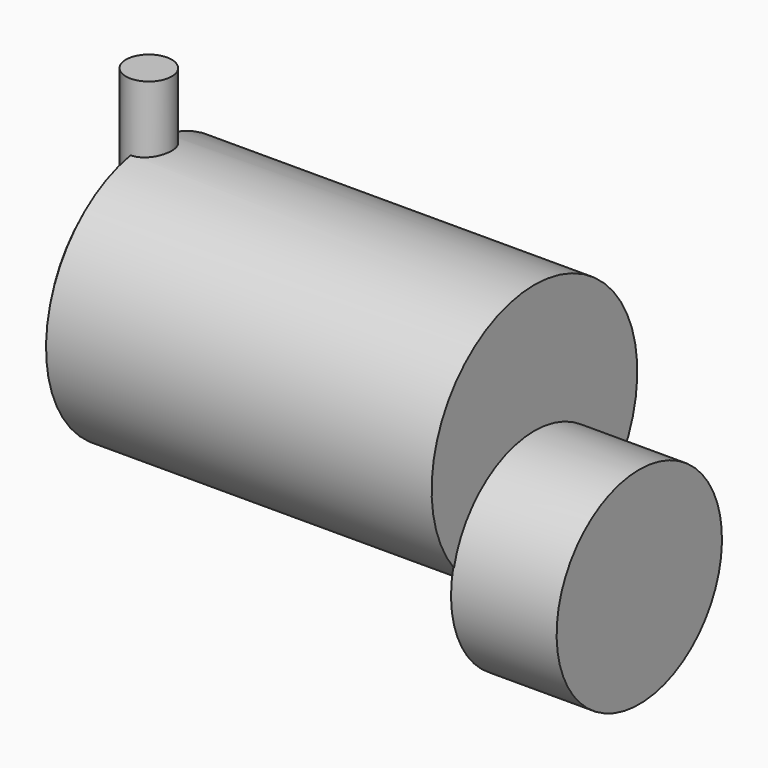
from build123d import *

# Parameters (mm, degrees)
F2_W = 54.2633533478
F2_H = 228.2263338566
F0_W = 914.4
F0_H = 304.8


# Not quite as in the source:
# - a feature names something its author has since deleted; it is built from what else it names


with BuildPart() as f3:
    # F2 (on Right) → F3 (revolve)
    with BuildSketch(Plane.YZ):
        with Locations((27.1316766739, 345.8204418421)):
            Rectangle(F2_W, F2_H)
    revolve(axis=Axis((0, 0, 345.8204418421), (0, 0, 1)))

    # F0 (on Front) → F4 (revolve)
    with BuildSketch(Plane.XZ):
        with BuildLine():
            Line((-118.2694360614, 0), (0, 0))
            Line((0, 0), (0, 304.8))
            ThreePointArc((0, 304.8), (-79.2984862526, 160.2240075344), (-118.2694360614, 0))
        make_face()
        with Locations((457.2, 152.4)):
            Rectangle(F0_W, F0_H)
    revolve(axis=Axis((457.2, 0, 0), (1, 0, 0)))

    # F1 (on face) → F5 (revolve)
    with BuildSketch(Plane.XZ):
        Polygon((914.4, 0), (912.6048088074, 0), (912.6048088074, -245.057374239), (1163.0200147629, -245.057374239), (1163.0200147629, 0), align=None)
    revolve(axis=Axis((1037.8124117851, 0, -245.057374239), (1, 0, 0)))


solid = f3.part
